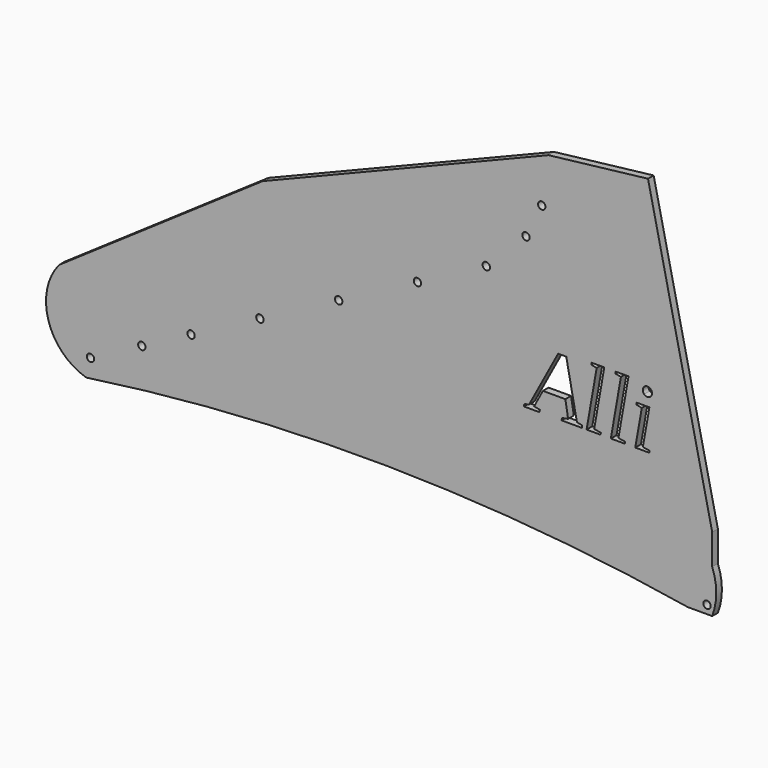
from build123d import *

# Parameters (mm, degrees)
F0_R     = 1.651
F1_DEPTH = 3.175


with BuildPart() as f1:
    # F0 (on Front) → F1 (new body)
    with BuildSketch(Plane.XZ):
        with BuildLine():
            Line((-91.7235008659, -10.6519622226), (-182.5513082058, -73.0949387128))
            ThreePointArc((-182.5513082058, -73.0949387128), (-187.3498879631, -96.5075485814), (-170.466153763, -113.4225179282))
            ThreePointArc((-170.466153763, -113.4225179282), (-36.1095650791, -104.4974979583), (98.0233131029, -116.3178149951))
            Line((98.0233131029, -116.3178149951), (108.933846237, -116.3178149951))
            ThreePointArc((108.933846237, -116.3178149951), (110.7304402005, -106.6101038659), (108.933846237, -96.9023927367))
            Line((108.933846237, -96.9023927367), (108.933846237, -83.3431183613))
            Line((108.933846237, -83.3431183613), (80.270888986, 46.2421850049))
            Line((80.270888986, 46.2421850049), (35.8280335171, 41.0442404951))
            Line((35.8280335171, 41.0442404951), (-91.7235008659, -10.6519622226))
        make_face()
        with Locations((-168.5793250799, -105.0686376895)):
            Circle(F0_R, mode=Mode.SUBTRACT)
        with Locations((-145.6571504202, -92.9395344899)):
            Circle(F0_R, mode=Mode.SUBTRACT)
        with Locations((-123.6779055701, -81.3093757901)):
            Circle(F0_R, mode=Mode.SUBTRACT)
        with Locations((-92.9428839156, -65.04616102)):
            Circle(F0_R, mode=Mode.SUBTRACT)
        with Locations((-57.7850724394, -46.4426589528)):
            Circle(F0_R, mode=Mode.SUBTRACT)
        with Locations((106.6226363182, -112.6031056046)):
            Circle(F0_R, mode=Mode.SUBTRACT)
        Polygon((29.4560794945, -59.7358805891), (32.0242086794, -60.2470721804), (31.8355546398, -61.2572841346), (24.8736120152, -61.2572841346), (25.0622660549, -60.2470721804), (27.1922310187, -59.7358805891), (40.1667604553, -35.5455642146), (43.7937865079, -35.5455642146), (48.5527367984, -59.7358805891), (50.9261263295, -60.2470721804), (50.7192154473, -61.2572841346), (41.6881640008, -61.2572841346), (41.895074883, -60.2470721804), (44.6153444225, -59.7358805891), (43.3982215861, -52.3783730427), (33.3569581853, -52.3783730427), align=None, mode=Mode.SUBTRACT)
        Polygon((60.760478848, -34.2310715512), (56.251038739, -59.9245346287), (59.2390753025, -60.3992125349), (59.0869349479, -61.2572841346), (52.8674372537, -61.2572841346), (57.3707917485, -35.5455642146), (54.9182892331, -35.0891431509), (55.0704295876, -34.2310715512), align=None, mode=Mode.SUBTRACT)
        Polygon((71.5807008641, -34.2310715512), (67.0712607551, -59.9245346287), (70.0592973185, -60.3992125349), (69.907156964, -61.2572841346), (63.6876592697, -61.2572841346), (68.1910137646, -35.5455642146), (65.7385112491, -35.0891431509), (65.8906516037, -34.2310715512), align=None, mode=Mode.SUBTRACT)
        Polygon((80.8977761772, -43.3777496671), (77.988852598, -59.9245346287), (80.9708035473, -60.3992125349), (80.8186631928, -61.2572841346), (74.5991654985, -61.2572841346), (77.5080890776, -44.7104991731), (75.0555865622, -44.2358212668), (75.2077269167, -43.3777496671), align=None, mode=Mode.SUBTRACT)
        with BuildLine():
            add(Edge.make_bspline(
                [(81.4637382961, -36.0750126484), (82.0722997143, -36.6835740667), (82.0722997143, -37.5416456664)],
                knots=[0, 0, 0, 1, 1, 1], degree=2))
            add(Edge.make_bspline(
                [(82.0722997143, -37.5416456664), (82.0722997143, -38.3814604235), (81.4637382961, -38.9900218417)],
                knots=[0, 0, 0, 1, 1, 1], degree=2))
            add(Edge.make_bspline(
                [(81.4637382961, -38.9900218417), (80.8551768779, -39.59858326), (80.0031908924, -39.59858326)],
                knots=[0, 0, 0, 1, 1, 1], degree=2))
            add(Edge.make_bspline(
                [(80.0031908924, -39.59858326), (79.1633761352, -39.59858326), (78.554814717, -38.9900218417)],
                knots=[0, 0, 0, 1, 1, 1], degree=2))
            add(Edge.make_bspline(
                [(78.554814717, -38.9900218417), (77.9462532988, -38.3814604235), (77.9462532988, -37.5416456664)],
                knots=[0, 0, 0, 1, 1, 1], degree=2))
            add(Edge.make_bspline(
                [(77.9462532988, -37.5416456664), (77.9462532988, -36.6835740667), (78.554814717, -36.0750126484)],
                knots=[0, 0, 0, 1, 1, 1], degree=2))
            add(Edge.make_bspline(
                [(78.554814717, -36.0750126484), (79.1633761352, -35.4664512302), (80.0031908924, -35.4664512302)],
                knots=[0, 0, 0, 1, 1, 1], degree=2))
            add(Edge.make_bspline(
                [(80.0031908924, -35.4664512302), (80.8551768779, -35.4664512302), (81.4637382961, -36.0750126484)],
                knots=[0, 0, 0, 1, 1, 1], degree=2))
        make_face(mode=Mode.SUBTRACT)
        with Locations((-22.6272609633, -27.8391568856)):
            Circle(F0_R, mode=Mode.SUBTRACT)
        with Locations((8.1077606912, -11.5759421154)):
            Circle(F0_R, mode=Mode.SUBTRACT)
        with Locations((25.8241575211, 5.8733294718)):
            Circle(F0_R, mode=Mode.SUBTRACT)
        with Locations((32.8517727122, 20.2778487448)):
            Circle(F0_R, mode=Mode.SUBTRACT)
    extrude(amount=F1_DEPTH)


solid = f1.part
